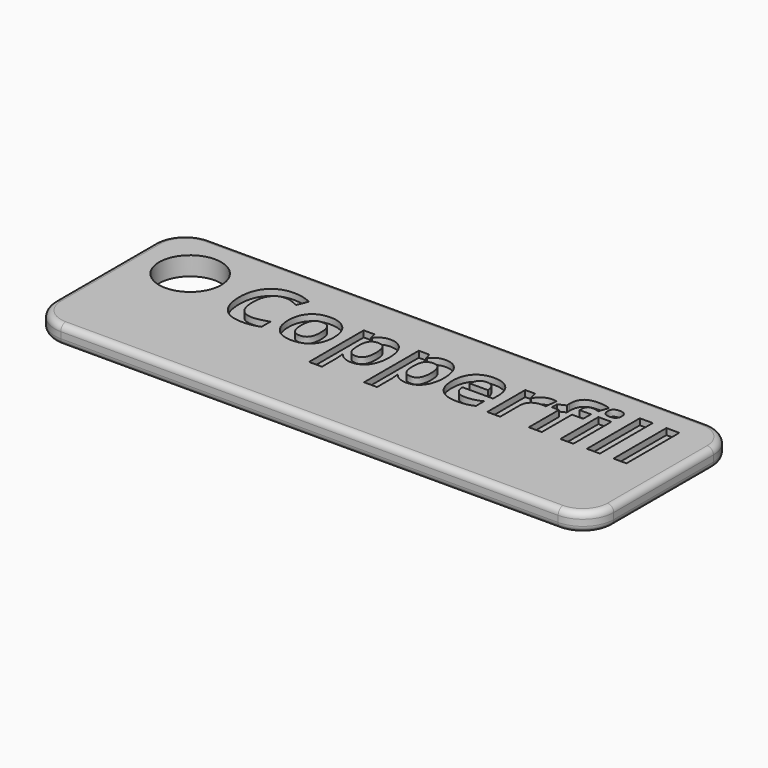
from build123d import *

# Parameters (mm, degrees)
F0_W         = 90
F0_H         = 30
F1_DEPTH     = 3
F2_R         = 1
F3_T3_ANGLE  = 90
F3_T6_ANGLE  = 90
F3_T9_ANGLE  = 90
F3_T12_ANGLE = 90
F3_T15_ANGLE = 90
F3_T18_ANGLE = 90
F3_T21_ANGLE = 90
F3_T24_ANGLE = 90
F3_T27_DEPTH = 3
F3_T30_DEPTH = 3
F3_T33_DEPTH = 3
F3_T36_DEPTH = 3
F4_R         = 5
F5_DEPTH     = 3
F6_TEXT_SIZE = 14.0025740026
F7_DEPTH     = 1


# Not quite as in the source:
# - a fillet or chamfer that OpenCascade refuses, or shapes differently, is made with other operations: its cross-section is extruded or revolved along the edge and cut away or added
# - Text() gives the source's letters only with a copy of the font that has no kerning and outlines rounded to 1/6400 em; it was checked with that copy


with BuildPart() as f1:
    # F0 (on Top) → F1 (new body)
    with BuildSketch(Plane.XY):
        Rectangle(F0_W, F0_H)
    extrude(amount=F1_DEPTH)

    # F2
    f2_edges = [f1.edges().sort_by_distance(p)[0] for p in [
        (0, 15, 3),
        (-45, 0, 3),
        (0, -15, 3),
        (45, 0, 3),
        (0, 15, 0),
        (-45, 0, 0),
        (0, -15, 0),
        (45, 0, 0),
    ]]
    fillet(f2_edges, radius=F2_R)

    # F3: fillet of radius 5 on 4 edges, made by hand


with BuildPart() as f3_tool1:
    # F3_s2 → F3_t3 (revolve)
    with BuildSketch(Plane.YZ.offset(-40.0001)):
        with BuildLine():
            ThreePointArc((-14.0001, 0), (-14.7072067812, 0.2928932188), (-15.0001, 1))
            Line((-15.0001, 1), (-15.0001, 0))
            Line((-15.0001, 0), (-14.0001, 0))
        make_face()
    revolve(axis=Axis((-40.0001, -10.0001, 0), (0, 0, -1)), revolution_arc=F3_T3_ANGLE)


with BuildPart() as f3_tool4:
    # F3_s5 → F3_t6 (revolve)
    with BuildSketch(Plane.XZ.offset(10.0001)):
        with BuildLine():
            ThreePointArc((-44.0001, 3), (-44.7072067812, 2.7071067812), (-45.0001, 2))
            Line((-45.0001, 2), (-45.0001, 3))
            Line((-45.0001, 3), (-44.0001, 3))
        make_face()
    revolve(axis=Axis((-40.0001, -10.0001, 3), (0, 0, 1)), revolution_arc=F3_T6_ANGLE)


with BuildPart() as f3_tool7:
    # F3_s8 → F3_t9 (revolve)
    with BuildSketch(Plane.XZ.offset(-10.0001)):
        with BuildLine():
            ThreePointArc((-44.0001, 0), (-44.7072067812, 0.2928932188), (-45.0001, 1))
            Line((-45.0001, 1), (-45.0001, 0))
            Line((-45.0001, 0), (-44.0001, 0))
        make_face()
    revolve(axis=Axis((-40.0001, 10.0001, 0), (0, 0, -1)), revolution_arc=F3_T9_ANGLE)


with BuildPart() as f3_tool10:
    # F3_s11 → F3_t12 (revolve)
    with BuildSketch(Plane.YZ.offset(-40.0001)):
        with BuildLine():
            ThreePointArc((14.0001, 3), (14.7072067812, 2.7071067812), (15.0001, 2))
            Line((15.0001, 2), (15.0001, 3))
            Line((15.0001, 3), (14.0001, 3))
        make_face()
    revolve(axis=Axis((-40.0001, 10.0001, 3), (0, 0, 1)), revolution_arc=F3_T12_ANGLE)


with BuildPart() as f3_tool13:
    # F3_s14 → F3_t15 (revolve)
    with BuildSketch(Plane.YZ.offset(40.0001)):
        with BuildLine():
            ThreePointArc((14.0001, 0), (14.7072067812, 0.2928932188), (15.0001, 1))
            Line((15.0001, 1), (15.0001, 0))
            Line((15.0001, 0), (14.0001, 0))
        make_face()
    revolve(axis=Axis((40.0001, 10.0001, 0), (0, 0, -1)), revolution_arc=F3_T15_ANGLE)


with BuildPart() as f3_tool16:
    # F3_s17 → F3_t18 (revolve)
    with BuildSketch(Plane.XZ.offset(-10.0001)):
        with BuildLine():
            ThreePointArc((44.0001, 3), (44.7072067812, 2.7071067812), (45.0001, 2))
            Line((45.0001, 2), (45.0001, 3))
            Line((45.0001, 3), (44.0001, 3))
        make_face()
    revolve(axis=Axis((40.0001, 10.0001, 3), (0, 0, 1)), revolution_arc=F3_T18_ANGLE)


with BuildPart() as f3_tool19:
    # F3_s20 → F3_t21 (revolve)
    with BuildSketch(Plane.XZ.offset(10.0001)):
        with BuildLine():
            ThreePointArc((44.0001, 0), (44.7072067812, 0.2928932188), (45.0001, 1))
            Line((45.0001, 1), (45.0001, 0))
            Line((45.0001, 0), (44.0001, 0))
        make_face()
    revolve(axis=Axis((40.0001, -10.0001, 0), (0, 0, -1)), revolution_arc=F3_T21_ANGLE)


with BuildPart() as f3_tool22:
    # F3_s23 → F3_t24 (revolve)
    with BuildSketch(Plane.YZ.offset(40.0001)):
        with BuildLine():
            ThreePointArc((-14.0001, 3), (-14.7072067812, 2.7071067812), (-15.0001, 2))
            Line((-15.0001, 2), (-15.0001, 3))
            Line((-15.0001, 3), (-14.0001, 3))
        make_face()
    revolve(axis=Axis((40.0001, -10.0001, 3), (0, 0, 1)), revolution_arc=F3_T24_ANGLE)


with BuildPart() as f3_tool25:
    # F3_s26 → F3_t27 (new body)
    with BuildSketch(Plane.XY):
        with BuildLine():
            ThreePointArc((45.0001, -10.0001), (43.5356339059, -13.5356339059), (40.0001, -15.0001))
            Line((40.0001, -15.0001), (40.0001, -15.1001))
            ThreePointArc((40.0001, -15.1001), (42.50005, -15.1), (45, -15.1))
            Line((45, -15.1), (45.1, -15))
            ThreePointArc((45.1, -15), (45.1, -12.50005), (45.1001, -10.0001))
            Line((45.1001, -10.0001), (45.0001, -10.0001))
        make_face()
    extrude(amount=F3_T27_DEPTH)


with BuildPart() as f3_tool28:
    # F3_s29 → F3_t30 (new body)
    with BuildSketch(Plane.XY):
        with BuildLine():
            ThreePointArc((40.0001, 15.0001), (43.5356339059, 13.5356339059), (45.0001, 10.0001))
            Line((45.0001, 10.0001), (45.1001, 10.0001))
            ThreePointArc((45.1001, 10.0001), (45.1, 12.50005), (45.1, 15))
            Line((45.1, 15), (45, 15.1))
            ThreePointArc((45, 15.1), (42.50005, 15.1), (40.0001, 15.1001))
            Line((40.0001, 15.1001), (40.0001, 15.0001))
        make_face()
    extrude(amount=F3_T30_DEPTH)


with BuildPart() as f3_tool31:
    # F3_s32 → F3_t33 (new body)
    with BuildSketch(Plane.XY):
        with BuildLine():
            ThreePointArc((-40.0001, 15.0001), (-43.5356339059, 13.5356339059), (-45.0001, 10.0001))
            Line((-45.0001, 10.0001), (-45.1001, 10.0001))
            ThreePointArc((-45.1001, 10.0001), (-45.1, 12.50005), (-45.1, 15))
            Line((-45.1, 15), (-45, 15.1))
            ThreePointArc((-45, 15.1), (-42.50005, 15.1), (-40.0001, 15.1001))
            Line((-40.0001, 15.1001), (-40.0001, 15.0001))
        make_face()
    extrude(amount=F3_T33_DEPTH)


with BuildPart() as f3_tool34:
    # F3_s35 → F3_t36 (new body)
    with BuildSketch(Plane.XY):
        with BuildLine():
            ThreePointArc((-45.0001, -10.0001), (-43.5356339059, -13.5356339059), (-40.0001, -15.0001))
            Line((-40.0001, -15.0001), (-40.0001, -15.1001))
            ThreePointArc((-40.0001, -15.1001), (-42.50005, -15.1), (-45, -15.1))
            Line((-45, -15.1), (-45.1, -15))
            ThreePointArc((-45.1, -15), (-45.1, -12.50005), (-45.1001, -10.0001))
            Line((-45.1001, -10.0001), (-45.0001, -10.0001))
        make_face()
    extrude(amount=F3_T36_DEPTH)


with BuildPart() as f1_1:
    add(f1.part)

    # F3_t37: cut F3_tool1, F3_tool4, F3_tool7, F3_tool10, F3_tool13, F3_tool16, F3_tool19, F3_tool22, F3_tool25, F3_tool28, F3_tool31, F3_tool34
    add([f3_tool1.part, f3_tool4.part, f3_tool7.part, f3_tool10.part, f3_tool13.part, f3_tool16.part, f3_tool19.part, f3_tool22.part, f3_tool25.part, f3_tool28.part, f3_tool31.part, f3_tool34.part], mode=Mode.SUBTRACT)

    # F4 (on face) → F5 (cut)
    with BuildSketch(Plane.XY.offset(3)):
        with Locations((-36, 6)):
            Circle(F4_R)
    extrude(amount=-F5_DEPTH, mode=Mode.SUBTRACT)

    # F6 (on face) → F7 (cut)
    with BuildSketch(Plane.XY.offset(3)):
        with Locations((-28, -0.0818532819)):
            Text('Copperfill', F6_TEXT_SIZE, font='Open Sans', font_style=FontStyle.BOLD, text_align=(TextAlign.LEFT, TextAlign.BOTTOM))
    extrude(amount=-F7_DEPTH, mode=Mode.SUBTRACT)


solid = f1_1.part
